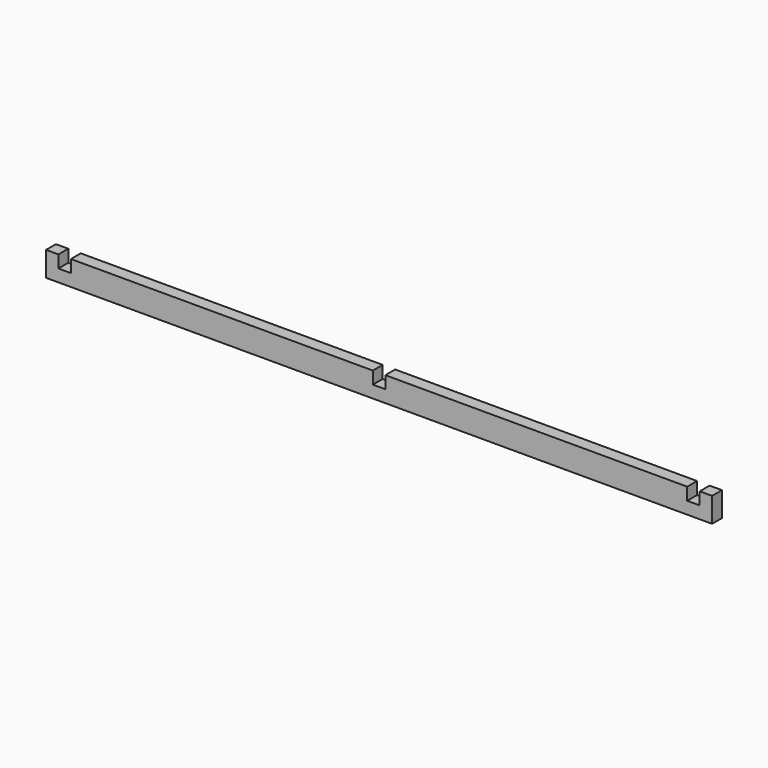
from build123d import *

# Parameters (mm, degrees)
F1_DEPTH = 3


# Not quite as in the source:
# - a feature names something its author has since deleted; it is built from what else it names


with BuildPart() as f1:
    # F0 (on Front) → F1 (new body)
    with BuildSketch(Plane.XZ):
        Polygon((-81.04, 6), (-81.04, 0), (81.04, 0), (81.04, 6), (78.04, 6), (78.04, 2.98), (75, 2.98), (75, 6), (1.52, 6), (1.52, 2.98), (-1.52, 2.98), (-1.52, 6), (-75, 6), (-75, 2.98), (-78.04, 2.98), (-78.04, 6), align=None)
    extrude(amount=F1_DEPTH)


solid = f1.part
